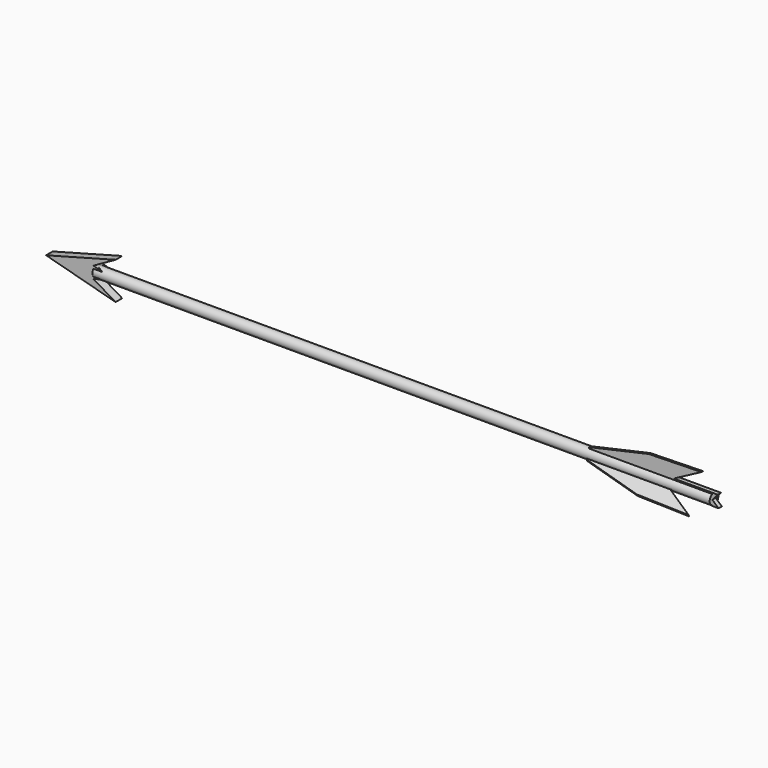
from build123d import *

# Parameters (mm, degrees)
F2_DEPTH      = 5.08
F3_DEPTH      = 5.08
F4_DEPTH      = 2.54
F5_COUNT      = 3
F6_DEPTH      = 10.16
F7_DEPTH      = 10.16
F8_DEPTH      = 7.62
F9_DEPTH      = 2.54
F9_DEPTH_BACK = 2.54


with BuildPart() as f1:
    # F0 (on Front) → F1 (revolve)
    with BuildSketch(Plane.XZ):
        Polygon((-531.0639472567, 0), (224.2752164602, 0), (184.5656899125, 6.6608362831), (-505.6800862797, 6.6608362831), align=None)
    revolve(axis=Axis((-140.7024349097, 0, 6.6608362831), (-1, 0, 0)))

    # F0 (on Front) → F2 (join)
    with BuildSketch(Plane.XZ):
        Polygon((-503.9185357909, -16.1311917064), (-531.0639472567, 0), (-505.6800862797, 6.6608362831), (-531.0639472567, 14.332789099), (-503.9185357909, 29.4528642727), (-588.9795422554, 6.6608362831), align=None)
    extrude(amount=F2_DEPTH)

    # F0 (on Front) → F3 (join)
    with BuildSketch(Plane.XZ):
        Polygon((-503.9185357909, -16.1311917064), (-531.0639472567, 0), (-505.6800862797, 6.6608362831), (-531.0639472567, 14.332789099), (-503.9185357909, 29.4528642727), (-588.9795422554, 6.6608362831), align=None)
    extrude(amount=-F3_DEPTH)



with BuildPart() as f4:
    # F0 (on Front) → F4 (new body)
    with BuildSketch(Plane.XZ):
        Polygon((138.8282477856, 14.332789099), (177.2306859493, 14.332789099), (210.8558267355, 32.1787036955), (146.4593857527, 30.6850112975), (73.320440948, 14.332789099), align=None)
    extrude(amount=F4_DEPTH)


with BuildPart() as f5_1:
    # F5: instance of F4
    add(f4.part.rotate(Axis((-140.7024349097, 0, 6.6608362831), (-1, 0, 0)), 1 * 360 / F5_COUNT))


with BuildPart() as f5_2:
    # F5: instance of F4
    add(f4.part.rotate(Axis((-140.7024349097, 0, 6.6608362831), (-1, 0, 0)), 2 * 360 / F5_COUNT))


with BuildPart() as f1_1:
    add(f1.part)
    # F6 (add): a face of the model
    f6_faces = [f5_1.part.faces().sort_by_distance(p)[0] for p in [
        (125.2755634487, 7.2791060352, 3.924712138),
    ]]

    add(f5_1.part)  # F6 merges F5_1
    extrude(f6_faces, amount=F6_DEPTH)

    # F7 (add): a face of the model
    f7_faces = [f4.part.faces().sort_by_distance(p)[0] for p in [
        (125.2755634487, -1.27, 14.332789099),
    ]]

    add(f4.part)  # F7 merges F4
    extrude(f7_faces, amount=F7_DEPTH)

    # F8 (add): a face of the model
    f8_faces = [f5_2.part.faces().sort_by_distance(p)[0] for p in [
        (125.2755634487, -6.0091060352, 1.7250076124),
    ]]

    add(f5_2.part)  # F8 merges F5_2
    extrude(f8_faces, amount=F8_DEPTH)

    # F0 (on Front) → F9 (join, two sides)
    with BuildSketch(Plane.XZ) as f9_sk:
        Polygon((184.5656899125, 6.6608362831), (224.2752164602, 6.6608362831), (230.9360527433, 14.332789099), (177.2306859493, 14.332789099), (138.8282477856, 14.332789099), align=None)
        Polygon((224.2752164602, 0), (231.9471692761, 0), (224.2752164602, 6.6608362831), (184.5656899125, 6.6608362831), align=None)
    extrude(amount=F9_DEPTH)
    extrude(f9_sk.sketch, amount=-F9_DEPTH_BACK)


solid = f1_1.part
